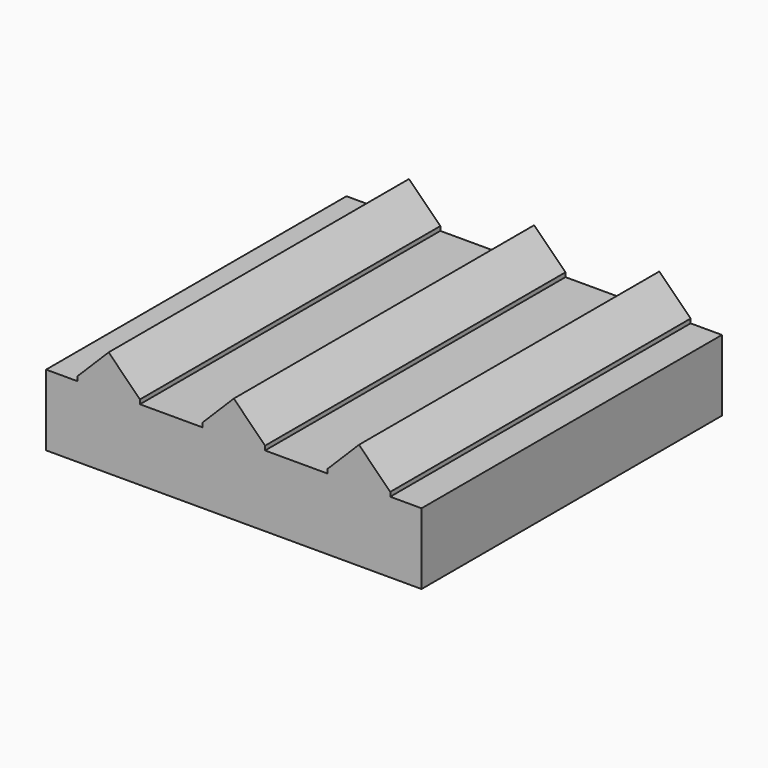
from build123d import *

# Parameters (mm, degrees)
F0_W     = 44
F0_H     = 44
F1_DEPTH = 25
F0_W_2   = 264
F0_H_2   = 264
F4_DEPTH = 50
F5_DEPTH = 44
F6_DEPTH = 22
F7_SIZE  = 21.99999


# Not quite as in the source:
# - a fillet or chamfer is up to 0.001 mm smaller than in the source, because OpenCascade refuses the exact size


with BuildPart() as f1:
    # F0 (on Top) → F1 (new body)
    with BuildSketch(Plane.XY):
        with Locations((-88, 88)):
            Rectangle(F0_W, F0_H)
    extrude(amount=F1_DEPTH)


with BuildPart() as f1b:
    # F0 (on Top) → F1, piece 2 (new body)
    with BuildSketch(Plane.XY):
        with Locations((0, 88)):
            Rectangle(F0_W, F0_H)
    extrude(amount=F1_DEPTH)


with BuildPart() as f1c:
    # F0 (on Top) → F1, piece 3 (new body)
    with BuildSketch(Plane.XY):
        Rectangle(F0_W, F0_H)
    extrude(amount=F1_DEPTH)


with BuildPart() as f1d:
    # F0 (on Top) → F1, piece 4 (new body)
    with BuildSketch(Plane.XY):
        with Locations((-88, 0)):
            Rectangle(F0_W, F0_H)
    extrude(amount=F1_DEPTH)


with BuildPart() as f2_1:
    # F2: instance of F1d
    add(f1d.part.mirror(Plane.YZ))


with BuildPart() as f2_2:
    # F2: instance of F1
    add(f1.part.mirror(Plane.YZ))


with BuildPart() as f3_1:
    # F3: instance of F1
    add(f1.part.mirror(Plane.XZ))


with BuildPart() as f3_2:
    # F3: instance of F1b
    add(f1b.part.mirror(Plane.XZ))


with BuildPart() as f3_3:
    # F3: instance of F2_2
    add(f2_2.part.mirror(Plane.XZ))


with BuildPart() as f1_1:
    add(f1.part)

    add(f1b.part)  # F4 merges F1b

    add(f1c.part)  # F4 merges F1c

    add(f1d.part)  # F4 merges F1d

    add(f2_1.part)  # F4 merges F2_1

    add(f2_2.part)  # F4 merges F2_2

    add(f3_1.part)  # F4 merges F3_1

    add(f3_2.part)  # F4 merges F3_2

    add(f3_3.part)  # F4 merges F3_3
    # F0 (on Top) → F4 (join)
    with BuildSketch(Plane.XY):
        Rectangle(F0_W_2, F0_H_2)
        with Locations((-88, 0)):
            Rectangle(F0_W, F0_H, mode=Mode.SUBTRACT)
        with Locations((-88, 88)):
            Rectangle(F0_W, F0_H, mode=Mode.SUBTRACT)
        Rectangle(F0_W, F0_H, mode=Mode.SUBTRACT)
        with Locations((0, 88)):
            Rectangle(F0_W, F0_H, mode=Mode.SUBTRACT)
        with Locations((-88, 0)):
            Rectangle(F0_W, F0_H)
        Rectangle(F0_W, F0_H)
        with Locations((-88, 88)):
            Rectangle(F0_W, F0_H)
        with Locations((0, 88)):
            Rectangle(F0_W, F0_H)
    extrude(amount=-F4_DEPTH)

    # F5 (add): faces of the model
    f5_faces = [f1_1.faces().sort_by_distance(p)[0] for p in [
        (-88, -66, 12.5),
        (-88, 22, 12.5),
        (0, 22, 12.5),
        (0, -66, 12.5),
        (88, -66, 12.5),
        (88, 22, 12.5),
    ]]
    extrude(f5_faces, amount=F5_DEPTH)

    # F6 (add, symmetric): faces of the model
    f6_faces = [f1_1.faces().sort_by_distance(p)[0] for p in [
        (-88, -110, 12.5),
        (0, -110, 12.5),
        (88, -110, 12.5),
        (-88, 110, 12.5),
        (0, 110, 12.5),
        (88, 110, 12.5),
    ]]
    extrude(f6_faces, amount=F6_DEPTH, both=True, dir=(0, -1, 0))

    # F7 (size 22 in the source; OpenCascade refuses exactly that, so slightly less here)
    f7_edges = [f1_1.edges().sort_by_distance(p)[0] for p in [
        (-110, 0, 25),
        (-66, 0, 25),
        (-22, 0, 25),
        (22, 0, 25),
        (110, 0, 25),
        (66, 0, 25),
    ]]
    chamfer(f7_edges, length=F7_SIZE)


solid = f1_1.part
